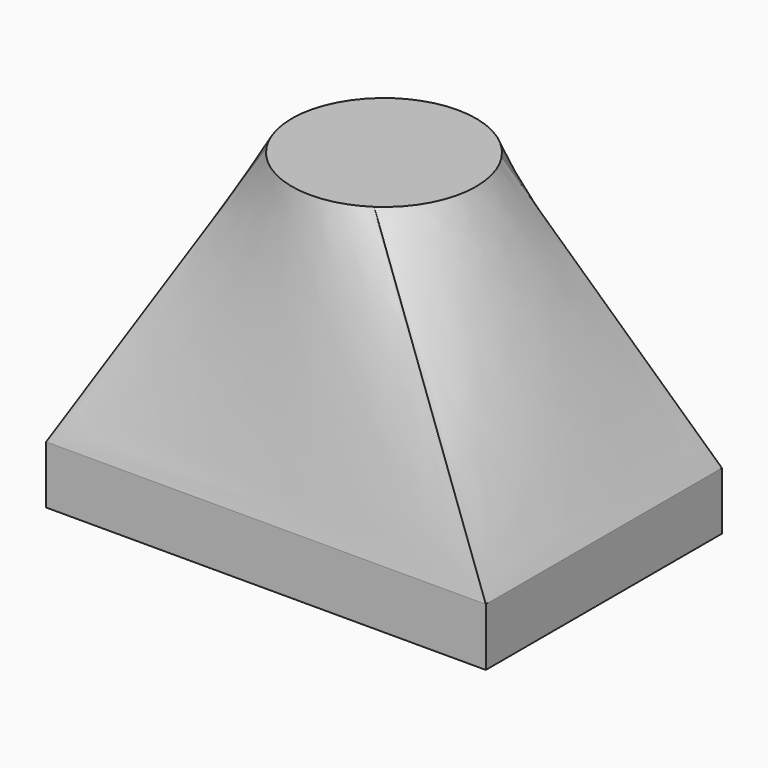
from build123d import *

# Parameters (mm, degrees)
F0_W      = 75.6886824965
F0_H      = 9.952143766
F1_DEPTH  = 25.4
F1_FACE_W = 75.6886824965
F1_FACE_H = 50.8


# Not quite as in the source:
# - the arcs of a loft's sections are written as splines that run evenly, so that the points pair up as in the source's solid


with BuildPart() as f1:
    # F0 (on Front) → F1 (new body, symmetric)
    with BuildSketch(Plane.XZ):
        Rectangle(F0_W, F0_H)
    extrude(amount=F1_DEPTH, both=True)

    # F3 (on offset) → F4 section 0
    with BuildSketch(Plane.XY.offset(50.8)):
        with BuildLine():
            add(Edge.make_bspline(
                [(13.172476733, 8.8409759024), (12.0151956936, 10.5652490746), (10.5155256838, 12.0587368806), (7.0574476007, 14.3590337045), (5.1004001334, 15.1649376538), (1.0252670866, 15.9667856178), (-1.0912151021, 15.9624141396), (-5.1630010474, 15.1437391601), (-7.1167027301, 14.3297577724), (-8.8409759024, 13.172476733)],
                knots=[0, 0, 0, 0, 0.25, 0.25, 0.5, 0.5, 0.75, 0.75, 1, 1, 1, 1], degree=3))
            add(Edge.make_bspline(
                [(-8.8409759024, 13.172476733), (-10.5652490746, 12.0151956936), (-12.0587368806, 10.5155256838), (-14.3590337045, 7.0574476007), (-15.1649376538, 5.1004001334), (-15.9667856178, 1.0252670866), (-15.9624141396, -1.0912151021), (-15.1437391601, -5.1630010474), (-14.3297577724, -7.1167027301), (-13.172476733, -8.8409759024)],
                knots=[0, 0, 0, 0, 0.25, 0.25, 0.5, 0.5, 0.75, 0.75, 1, 1, 1, 1], degree=3))
            add(Edge.make_bspline(
                [(-13.172476733, -8.8409759024), (-12.0151956936, -10.5652490746), (-10.5155256838, -12.0587368806), (-7.0574476007, -14.3590337045), (-5.1004001334, -15.1649376538), (-1.0252670866, -15.9667856178), (1.0912151021, -15.9624141396), (5.1630010474, -15.1437391601), (7.1167027301, -14.3297577724), (8.8409759024, -13.172476733)],
                knots=[0, 0, 0, 0, 0.25, 0.25, 0.5, 0.5, 0.75, 0.75, 1, 1, 1, 1], degree=3))
            add(Edge.make_bspline(
                [(8.8409759024, -13.172476733), (10.5652490746, -12.0151956936), (12.0587368806, -10.5155256838), (14.3590337045, -7.0574476007), (15.1649376538, -5.1004001334), (15.9667856178, -1.0252670866), (15.9624141396, 1.0912151021), (15.1437391601, 5.1630010474), (14.3297577724, 7.1167027301), (13.172476733, 8.8409759024)],
                knots=[0, 0, 0, 0, 0.25, 0.25, 0.5, 0.5, 0.75, 0.75, 1, 1, 1, 1], degree=3))
        make_face()
    # F1_face (on face) → F4 section 1
    with BuildSketch(Plane.XY.offset(4.976071883)):
        Rectangle(F1_FACE_W, F1_FACE_H)
    loft(ruled=True)


solid = f1.part
